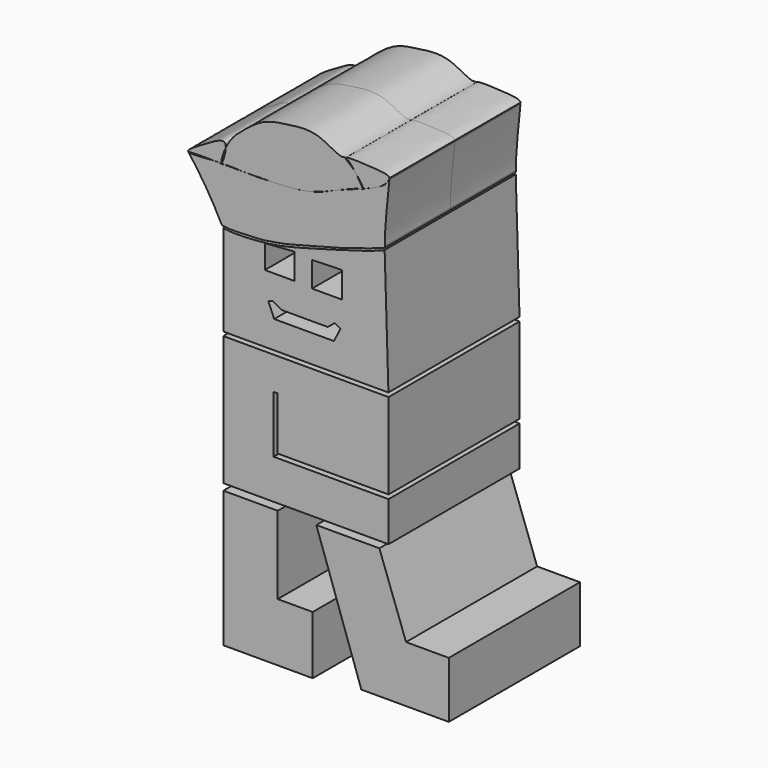
from build123d import *

# Parameters (mm, degrees)
F1_DEPTH      = 12.7
F1_DEPTH_BACK = 12.7


# Not quite as in the source:
# - a feature names something its author has since deleted; it is built from what else it names


with BuildPart() as f1:
    # F0 (on Front) → F1 (new body, two sides)
    with BuildSketch(Plane.XZ) as f1_sk:
        with BuildLine():
            add(Edge.make_bspline(
                [(-88.6765941978, 24.2591518909), (-88.676181883, 24.2590005668), (-88.6757689839, 24.2588493472), (-88.6753555008, 24.2586982322)],
                knots=[0, 0, 0, 0, 4.59815e-05, 4.59815e-05, 4.59815e-05, 4.59815e-05], degree=3))
            Line((-88.6765941978, 24.2591518909), (-88.6765941978, 10.1100709289))
            Line((-88.6765941978, 10.1100709289), (-63.0800493449, 10.1100709289))
            Line((-63.0800493449, 10.1100709289), (-63.6637075159, 29.3709366794))
            Line((-63.6637075159, 29.3709366794), (-64.1699039165, 29.1051819762))
            Line((-64.1699039165, 29.1051819762), (-64.7639196973, 28.9203976704))
            Line((-64.7639196973, 28.9203976704), (-65.5745303374, 28.6319091556))
            Line((-65.5745303374, 28.6319091556), (-67.1760400873, 28.1224887458))
            Line((-67.1760400873, 28.1224887458), (-68.6502717975, 27.6911423607))
            add(Edge.make_bspline(
                [(-70.894030415, 27.0381318624), (-70.1317684635, 27.256307302), (-69.3736818752, 27.476571284), (-68.6502717975, 27.6911423607)],
                knots=[0.2279945979, 0.2279945979, 0.2279945979, 0.2279945979, 0.247245534, 0.247245534, 0.247245534, 0.247245534], degree=3))
            add(Edge.make_bspline(
                [(-72.906285927, 26.4692383245), (-72.246354557, 26.6536394297), (-71.5685577228, 26.8450679274), (-70.894030415, 27.0381318624)],
                knots=[0.2109594015, 0.2109594015, 0.2109594015, 0.2109594015, 0.2279945979, 0.2279945979, 0.2279945979, 0.2279945979], degree=3))
            add(Edge.make_bspline(
                [(-74.0934775144, 26.1396786733), (-73.707677612, 26.2460726704), (-73.3103302266, 26.3563383796), (-72.906285927, 26.4692383245)],
                knots=[0.2005295684, 0.2005295684, 0.2005295684, 0.2005295684, 0.2109594015, 0.2109594015, 0.2109594015, 0.2109594015], degree=3))
            Line((-74.0934775144, 26.1396786733), (-75.0365182757, 25.8767232299))
            Line((-75.0365182757, 25.8767232299), (-75.7828429341, 25.6783552468))
            add(Edge.make_bspline(
                [(-76.5956836697, 25.4603034028), (-76.3368763961, 25.5291025193), (-76.0665517581, 25.6016964009), (-75.7828429341, 25.6783552468)],
                knots=[0.1756550657, 0.1756550657, 0.1756550657, 0.1756550657, 0.1843973599, 0.1843973599, 0.1843973599, 0.1843973599], degree=3))
            add(Edge.make_bspline(
                [(-77.3195936734, 25.2701518586), (-77.0880330237, 25.3301143771), (-76.8473015317, 25.3934154581), (-76.5956836697, 25.4603034028)],
                knots=[0.1671556239, 0.1671556239, 0.1671556239, 0.1671556239, 0.1756550657, 0.1756550657, 0.1756550657, 0.1756550657], degree=3))
            add(Edge.make_bspline(
                [(-78.2819622434, 25.0277422611), (-77.9772068237, 25.1019241231), (-77.6582053854, 25.1824685192), (-77.3195936734, 25.2701518586)],
                knots=[0.154726869, 0.154726869, 0.154726869, 0.154726869, 0.1671556239, 0.1671556239, 0.1671556239, 0.1671556239], degree=3))
            add(Edge.make_bspline(
                [(-79.7086635234, 24.7069066365), (-79.2560431416, 24.7986404801), (-78.7886960811, 24.9043959408), (-78.2819622434, 25.0277422611)],
                knots=[0.1340608848, 0.1340608848, 0.1340608848, 0.1340608848, 0.154726869, 0.154726869, 0.154726869, 0.154726869], degree=3))
            add(Edge.make_bspline(
                [(-80.8770336189, 24.4963051116), (-80.4878603762, 24.557399363), (-80.1038758883, 24.6268078368), (-79.7086635234, 24.7069066365)],
                knots=[0.1160160667, 0.1160160667, 0.1160160667, 0.1160160667, 0.1340608848, 0.1340608848, 0.1340608848, 0.1340608848], degree=3))
            Line((-80.8770336189, 24.4963051116), (-80.9098272944, 24.4904190618))
            Line((-80.9098272944, 24.4904190618), (-81.33696908, 24.4221940953))
            Line((-81.33696908, 24.4221940953), (-82.0637136126, 24.3332062233))
            Line((-82.0637136126, 24.3332062233), (-82.8794404293, 24.2501490134))
            Line((-82.8794404293, 24.2501490134), (-83.6002468491, 24.1937909592))
            Line((-83.6002468491, 24.1937909592), (-83.8359130376, 24.1790783462))
            add(Edge.make_bspline(
                [(-84.4445790934, 24.1410793947), (-84.2406040529, 24.1525204663), (-84.0370967315, 24.1652457772), (-83.8359130376, 24.1790783462)],
                knots=[0.0668457733, 0.0668457733, 0.0668457733, 0.0668457733, 0.0744285702, 0.0744285702, 0.0744285702, 0.0744285702], degree=3))
            Line((-84.4445790934, 24.1410793947), (-85.147680285, 24.0971848685))
            Line((-85.147680285, 24.0971848685), (-85.6315054246, 24.0900506289))
            add(Edge.make_bspline(
                [(-86.6028345544, 24.0757279031), (-86.2940429361, 24.0752792341), (-85.9672821173, 24.0803380751), (-85.6315054246, 24.0900506289)],
                knots=[0.0392199906, 0.0392199906, 0.0392199906, 0.0392199906, 0.0520326334, 0.0520326334, 0.0520326334, 0.0520326334], degree=3))
            add(Edge.make_bspline(
                [(-87.4198373818, 24.0923570373), (-87.1684176734, 24.0814558229), (-86.8935919097, 24.0761503687), (-86.6028345544, 24.0757279031)],
                knots=[0.0271556406, 0.0271556406, 0.0271556406, 0.0271556406, 0.0392199906, 0.0392199906, 0.0392199906, 0.0392199906], degree=3))
            add(Edge.make_bspline(
                [(-88.0641563934, 24.1389165741), (-87.8745442647, 24.1179875567), (-87.6576624685, 24.1026688074), (-87.4198373818, 24.0923570373)],
                knots=[0.0157436273, 0.0157436273, 0.0157436273, 0.0157436273, 0.0271556406, 0.0271556406, 0.0271556406, 0.0271556406], degree=3))
            add(Edge.make_bspline(
                [(-88.5565382268, 24.2221505155), (-88.4259838036, 24.1880082148), (-88.2595489318, 24.1604836219), (-88.0641563934, 24.1389165741)],
                knots=[0.0039837136, 0.0039837136, 0.0039837136, 0.0039837136, 0.0157436273, 0.0157436273, 0.0157436273, 0.0157436273], degree=3))
            add(Edge.make_bspline(
                [(-88.6359078797, 24.2451631992), (-88.6111654233, 24.237180281), (-88.5846857461, 24.2295115917), (-88.5565382268, 24.2221505155)],
                knots=[0.0014482776, 0.0014482776, 0.0014482776, 0.0014482776, 0.0039837136, 0.0039837136, 0.0039837136, 0.0039837136], degree=3))
            Line((-88.6359078797, 24.2451631992), (-88.6737406254, 24.2561325431))
            Line((-88.6737406254, 24.2561325431), (-88.6753555008, 24.2586982322))
        make_face()
        Polygon((-82.2262391448, 20.598737523), (-82.2262391448, 24.2591518909), (-77.6218995452, 24.6051102877), (-77.6218995452, 20.598737523), align=None, mode=Mode.SUBTRACT)
        Polygon((-80.7911232114, 14.3798924983), (-81.6880688071, 16.5325701237), (-80.9705108404, 16.7717561126), (-79.6549841762, 15.994399786), (-72.4793970585, 15.994399786), (-71.4150190353, 16.8674312532), (-70.5061107874, 16.4129771292), (-71.5226531029, 14.3798924983), align=None, mode=Mode.SUBTRACT)
        Polygon((-74.9200507998, 20.4430520535), (-74.9200507998, 24.3614321552), (-70.2414959669, 24.4861954051), (-70.2414959669, 20.4478651285), align=None, mode=Mode.SUBTRACT)
    extrude(amount=F1_DEPTH)
    extrude(f1_sk.sketch, amount=-F1_DEPTH_BACK)


with BuildPart() as f1b:
    # F0 (on Front) → F1, piece 2 (new body, two sides)
    with BuildSketch(Plane.XZ) as f1_2_sk:
        with BuildLine():
            Line((-89.1806710013, 25.0642394208), (-88.8575675001, 24.5481938542))
            Line((-88.8575675001, 24.5481938542), (-87.680645287, 24.4102943689))
            Line((-87.680645287, 24.4102943689), (-86.5415930748, 24.4221594185))
            Line((-86.5415930748, 24.4221594185), (-85.2364301682, 24.4696196169))
            Line((-85.2364301682, 24.4696196169), (-83.563439548, 24.5289467275))
            Line((-83.563439548, 24.5289467275), (-82.4006572366, 24.6238671243))
            Line((-82.4006572366, 24.6238671243), (-81.1148583889, 24.827260524))
            Line((-81.1148583889, 24.827260524), (-80.175191164, 24.9782800674))
            Line((-80.175191164, 24.9782800674), (-78.8160189986, 25.246758014))
            Line((-78.8160189986, 25.246758014), (-77.2387161851, 25.6494730711))
            Line((-77.2387161851, 25.6494730711), (-75.208351016, 26.1864289641))
            Line((-75.208351016, 26.1864289641), (-73.3753862668, 26.6711798054))
            Line((-73.3753862668, 26.6711798054), (-70.5099925399, 27.4281390011))
            Line((-70.5099925399, 27.4281390011), (-68.3453977108, 28.0993320048))
            Line((-68.3453977108, 28.0993320048), (-65.8955350518, 28.871204704))
            Line((-65.8955350518, 28.871204704), (-63.6414005769, 29.6839251888))
            Line((-63.6414005769, 29.6839251888), (-63.6204607901, 29.9628862484))
            add(Edge.make_bspline(
                [(-63.6204607901, 29.9628862484), (-63.7690930896, 31.4681703482), (-63.0734122524, 37.8136935829), (-62.9346598656, 39.1672787688)],
                knots=[0.3407241659, 0.3407241659, 0.3407241659, 0.3407241659, 0.4433037601, 0.4433037601, 0.4433037601, 0.4433037601], degree=3))
            add(Edge.make_bspline(
                [(-62.9346598656, 39.1672787688), (-62.99116387, 39.0074353898), (-63.1238176876, 38.8255438406), (-63.3057207132, 38.6381461886)],
                knots=[0.3858068106, 0.3858068106, 0.3858068106, 0.3858068106, 0.4313082922, 0.4313082922, 0.4313082922, 0.4313082922], degree=3))
            add(Edge.make_bspline(
                [(-63.3057207132, 38.6381461886), (-63.591865805, 38.282485153), (-64.0700130065, 37.9519174396), (-64.6626520258, 37.6396269978)],
                knots=[0.4854255945, 0.4854255945, 0.4854255945, 0.4854255945, 0.5132501123, 0.5132501123, 0.5132501123, 0.5132501123], degree=3))
            add(Edge.make_bspline(
                [(-64.6626520258, 37.6396269978), (-64.9284082914, 37.492687811), (-65.1932928871, 37.3699325807), (-65.4429785447, 37.2647073069)],
                knots=[0.5161566053, 0.5161566053, 0.5161566053, 0.5161566053, 0.5606076079, 0.5606076079, 0.5606076079, 0.5606076079], degree=3))
            add(Edge.make_bspline(
                [(-65.4429785447, 37.2647073069), (-65.8563362693, 37.081501475), (-66.3008735293, 36.9041305775), (-66.7586636583, 36.7310181908)],
                knots=[0.5246441776, 0.5246441776, 0.5246441776, 0.5246441776, 0.5417236467, 0.5417236467, 0.5417236467, 0.5417236467], degree=3))
            add(Edge.make_bspline(
                [(-66.7586636583, 36.7310181908), (-66.8712838712, 36.6647105624), (-66.9239643529, 36.6009277441), (-66.9972679395, 36.641578996)],
                knots=[0.6640545001, 0.6640545001, 0.6640545001, 0.6640545001, 0.7134494162, 0.7134494162, 0.7134494162, 0.7134494162], degree=3))
            add(Edge.make_bspline(
                [(-66.9972679395, 36.641578996), (-67.0125383393, 36.5119331388), (-67.1907492056, 36.5231425104), (-67.4698356723, 36.4682586449)],
                knots=[0.5691718068, 0.5691718068, 0.5691718068, 0.5691718068, 0.5952228955, 0.5952228955, 0.5952228955, 0.5952228955], degree=3))
            add(Edge.make_bspline(
                [(-67.4698356723, 36.4682586449), (-68.3929391768, 36.1336333741), (-69.5493172224, 35.7381934495), (-70.5194605701, 35.3447298383), (-70.696805174, 35.2710997008)],
                knots=[0.5504682125, 0.5504682125, 0.5504682125, 0.5504682125, 0.5842531146, 0.5920722335, 0.5920722335, 0.5920722335, 0.5920722335], degree=3))
            add(Edge.make_bspline(
                [(-70.696805174, 35.2710997008), (-70.908839023, 35.1812273665), (-71.1199071334, 35.0913269662), (-71.3269268074, 35.0033066073)],
                knots=[0.6590265835, 0.6590265835, 0.6590265835, 0.6590265835, 0.6698079497, 0.6698079497, 0.6698079497, 0.6698079497], degree=3))
            add(Edge.make_bspline(
                [(-71.3269268074, 35.0033066073), (-72.6834973217, 34.4164241105), (-73.8406974955, 33.8702485293), (-75.6439072937, 33.4965059757)],
                knots=[0.6016179317, 0.6016179317, 0.6016179317, 0.6016179317, 0.6649272201, 0.6649272201, 0.6649272201, 0.6649272201], degree=3))
            add(Edge.make_bspline(
                [(-75.6439072937, 33.4965059757), (-76.405580982, 33.3335271633), (-77.2236332809, 33.2252564375), (-78.0591693269, 33.1491839613)],
                knots=[0.7483248245, 0.7483248245, 0.7483248245, 0.7483248245, 0.7877632518, 0.7877632518, 0.7877632518, 0.7877632518], degree=3))
            add(Edge.make_bspline(
                [(-78.0591693269, 33.1491839613), (-78.9314375594, 33.0688250448), (-79.9140408829, 33.0151128871), (-80.9525646713, 32.9802233287)],
                knots=[0.6892796952, 0.6892796952, 0.6892796952, 0.6892796952, 0.7121210529, 0.7121210529, 0.7121210529, 0.7121210529], degree=3))
            add(Edge.make_bspline(
                [(-80.9525646713, 32.9802233287), (-82.6104794056, 32.9162984037), (-84.1581399366, 32.8778860173), (-85.6189520723, 32.9232138611)],
                knots=[0.8331267481, 0.8331267481, 0.8331267481, 0.8331267481, 0.912449519, 0.912449519, 0.912449519, 0.912449519], degree=3))
            add(Edge.make_bspline(
                [(-85.6189520723, 32.9232138611), (-86.594573022, 32.9259699322), (-87.5521865291, 32.9348252964), (-88.4524292433, 32.944119984)],
                knots=[0.744974607, 0.744974607, 0.744974607, 0.744974607, 0.7654790219, 0.7654790219, 0.7654790219, 0.7654790219], degree=3))
            add(Edge.make_bspline(
                [(-88.4524292433, 32.944119984), (-88.7063087421, 32.9022333853), (-88.8776467113, 32.8279592391), (-88.9438291909, 32.9492656946)],
                knots=[0.9742592774, 0.9742592774, 0.9742592774, 0.9742592774, 1, 1, 1, 1], degree=3))
            add(Edge.make_bspline(
                [(-88.9438291909, 32.9492656946), (-89.0352585897, 32.8295840724), (-89.0788010883, 32.9176528435), (-89.3225391675, 32.9532516827)],
                knots=[0.6558803024, 0.6558803024, 0.6558803024, 0.6558803024, 0.7317333454, 0.7317333454, 0.7317333454, 0.7317333454], degree=3))
            add(Edge.make_bspline(
                [(-89.3225391675, 32.9532516827), (-89.5940767888, 32.9560898012), (-89.8585710886, 32.9587851097), (-90.1147749683, 32.9611582906)],
                knots=[0.7722377312, 0.7722377312, 0.7722377312, 0.7722377312, 0.7787258229, 0.7787258229, 0.7787258229, 0.7787258229], degree=3))
            add(Edge.make_bspline(
                [(-90.1147749683, 32.9611582906), (-91.4362647143, 32.8979274564), (-93.6540192513, 32.6111194745), (-94.0586850047, 32.8551717103)],
                knots=[0.7863292069, 0.7863292069, 0.7863292069, 0.7863292069, 1, 1, 1, 1], degree=3))
            Line((-94.0586850047, 32.8551717103), (-93.7775747638, 32.4061957846))
            add(Edge.make_bspline(
                [(-93.7775747638, 32.4061957846), (-92.6941800923, 31.2024334146), (-89.8309867411, 26.6093738398), (-89.1806710013, 25.0642394208)],
                knots=[0.858322558, 0.858322558, 0.858322558, 0.858322558, 0.9647554778, 0.9647554778, 0.9647554778, 0.9647554778], degree=3))
        make_face()
    extrude(amount=F1_DEPTH)
    extrude(f1_2_sk.sketch, amount=-F1_DEPTH_BACK)


with BuildPart() as f1c:
    # F0 (on Front) → F1, piece 3 (new body, two sides)
    with BuildSketch(Plane.XZ) as f1_3_sk:
        Polygon((-63.0613416433, 9.4927120954), (-88.6765941978, 9.4927120954), (-88.6765941978, 0), (-88.6765941978, -10.5822533369), (-63.0613416433, -10.5822533369), (-63.0613416433, -4.4350544922), (-80.8818116784, -4.4350544922), (-80.8818116784, 4.4147078879), (-80.3020894527, 4.4147078879), (-80.3020894527, -3.7941283081), (-63.0613416433, -3.7941283081), align=None)
    extrude(amount=F1_DEPTH)
    extrude(f1_3_sk.sketch, amount=-F1_DEPTH_BACK)


with BuildPart() as f1d:
    # F0 (on Front) → F1, piece 4 (new body, two sides)
    with BuildSketch(Plane.XZ) as f1_4_sk:
        with BuildLine():
            add(Edge.make_bspline(
                [(-94.0586850047, 32.8551717103), (-94.4654065338, 33.1004637757), (-91.5178597494, 34.7172704345), (-88.4386957073, 36.6762673441), (-88.2852047026, 35.5322981305), (-88.2893016676, 35.317583748)],
                knots=[0, 0, 0, 0, 0.2147562796, 0.444264687, 0.4880842191, 0.4880842191, 0.4880842191, 0.4880842191], degree=3))
            add(Edge.make_bspline(
                [(-90.1147749683, 32.9611582906), (-92.2185943193, 32.9806456768), (-93.7634005143, 32.9784123854), (-94.0586850047, 32.8551717103)],
                knots=[0.7787258229, 0.7787258229, 0.7787258229, 0.7787258229, 0.8320028174, 0.8320028174, 0.8320028174, 0.8320028174], degree=3))
            add(Edge.make_bspline(
                [(-89.3225391675, 32.9532516827), (-89.4979716868, 32.9788742447), (-89.7771159455, 32.9773146488), (-90.1147749683, 32.9611582906)],
                knots=[0.7317333454, 0.7317333454, 0.7317333454, 0.7317333454, 0.7863292069, 0.7863292069, 0.7863292069, 0.7863292069], degree=3))
            add(Edge.make_bspline(
                [(-88.9438291909, 32.9492656946), (-89.0714727093, 32.9506129158), (-89.1977497163, 32.9519473801), (-89.3225391675, 32.9532516827)],
                knots=[0.7692560251, 0.7692560251, 0.7692560251, 0.7692560251, 0.7722377312, 0.7722377312, 0.7722377312, 0.7722377312], degree=3))
            add(Edge.make_bspline(
                [(-88.9438291909, 32.9492656946), (-89.0819981393, 33.2025167887), (-88.7618492252, 34.3082015855), (-88.2893016589, 35.3175837458)],
                knots=[0, 0, 0, 0, 0.0537388232, 0.0537388232, 0.0537388232, 0.0537388232], degree=3))
        make_face()
    extrude(amount=F1_DEPTH)
    extrude(f1_4_sk.sketch, amount=-F1_DEPTH_BACK)


with BuildPart() as f1e:
    # F0 (on Front) → F1, piece 5 (new body, two sides)
    with BuildSketch(Plane.XZ) as f1_5_sk:
        with BuildLine():
            add(Edge.make_bspline(
                [(-88.2893016589, 35.3175837458), (-88.1899717612, 35.5297567288), (-87.4282788512, 37.0229144843), (-85.6108289308, 38.5700062743), (-82.4464479, 41.1116553012), (-78.4456250447, 41.644345132), (-74.1132724556, 42.2162050244), (-70.5326189415, 39.6499089464), (-69.9159322613, 40.020232556), (-69.6954354644, 39.9633795023)],
                knots=[0.0537388232, 0.0537388232, 0.0537388232, 0.0537388232, 0.0650347692, 0.1348604038, 0.2069273895, 0.2800852866, 0.3577229921, 0.4305213633, 0.4616432126, 0.4616432126, 0.4616432126, 0.4616432126], degree=3))
            add(Edge.make_bspline(
                [(-88.2893016676, 35.317583748), (-88.3049899843, 34.495388012), (-88.7415763291, 33.2140158836), (-88.9438291909, 32.9492656946)],
                knots=[0.4880842191, 0.4880842191, 0.4880842191, 0.4880842191, 0.6558803024, 0.6558803024, 0.6558803024, 0.6558803024], degree=3))
            add(Edge.make_bspline(
                [(-88.4524292433, 32.944119984), (-88.6182578996, 32.9458321062), (-88.7821398929, 32.9475591352), (-88.9438291909, 32.9492656946)],
                knots=[0.7654790219, 0.7654790219, 0.7654790219, 0.7654790219, 0.7692560251, 0.7692560251, 0.7692560251, 0.7692560251], degree=3))
            add(Edge.make_bspline(
                [(-85.6189520723, 32.9232138611), (-86.7572436907, 32.9585341486), (-87.8428025932, 33.0446999322), (-88.4524292433, 32.944119984)],
                knots=[0.912449519, 0.912449519, 0.912449519, 0.912449519, 0.9742592774, 0.9742592774, 0.9742592774, 0.9742592774], degree=3))
            add(Edge.make_bspline(
                [(-80.9525646713, 32.9802233287), (-82.446311143, 32.9300404101), (-84.0557465065, 32.9187978983), (-85.6189520723, 32.9232138611)],
                knots=[0.7121210529, 0.7121210529, 0.7121210529, 0.7121210529, 0.744974607, 0.744974607, 0.744974607, 0.744974607], degree=3))
            add(Edge.make_bspline(
                [(-78.0591693269, 33.1491839613), (-79.0202329114, 33.0616826656), (-80.00442824, 33.0167810292), (-80.9525646713, 32.9802233287)],
                knots=[0.7877632518, 0.7877632518, 0.7877632518, 0.7877632518, 0.8331267481, 0.8331267481, 0.8331267481, 0.8331267481], degree=3))
            add(Edge.make_bspline(
                [(-75.6439072937, 33.4965059757), (-76.2263444498, 33.3757870498), (-77.0002283612, 33.2534476063), (-77.9100997071, 33.1629172061), (-78.0591693269, 33.1491839613)],
                knots=[0.6649272201, 0.6649272201, 0.6649272201, 0.6649272201, 0.685376134, 0.6892796952, 0.6892796952, 0.6892796952, 0.6892796952], degree=3))
            add(Edge.make_bspline(
                [(-71.3269268074, 35.0033066073), (-72.8345778324, 34.3622854825), (-74.1275122007, 33.8209759885), (-75.6439072937, 33.4965059757)],
                knots=[0.6698079497, 0.6698079497, 0.6698079497, 0.6698079497, 0.7483248245, 0.7483248245, 0.7483248245, 0.7483248245], degree=3))
            add(Edge.make_bspline(
                [(-70.696805174, 35.2710997008), (-70.9133101386, 35.1812109195), (-71.1223847401, 35.0917960429), (-71.3269268074, 35.0033066073)],
                knots=[0.5920722335, 0.5920722335, 0.5920722335, 0.5920722335, 0.6016179317, 0.6016179317, 0.6016179317, 0.6016179317], degree=3))
            add(Edge.make_bspline(
                [(-67.4698356723, 36.4682586449), (-68.1533674068, 36.3338384266), (-69.4419974553, 35.8029605303), (-70.696805174, 35.2710997008)],
                knots=[0.5952228955, 0.5952228955, 0.5952228955, 0.5952228955, 0.6590265835, 0.6590265835, 0.6590265835, 0.6590265835], degree=3))
            add(Edge.make_bspline(
                [(-66.9972679395, 36.641578996), (-67.1538562949, 36.5833678168), (-67.3116117825, 36.5256148479), (-67.4698356723, 36.4682586449)],
                knots=[0.5446773358, 0.5446773358, 0.5446773358, 0.5446773358, 0.5504682125, 0.5504682125, 0.5504682125, 0.5504682125], degree=3))
            add(Edge.make_bspline(
                [(-66.9972679395, 36.641578996), (-67.1899806678, 36.7484498059), (-67.5252293414, 37.5771134318), (-68.0491964268, 38.2991926754)],
                knots=[0.7134494162, 0.7134494162, 0.7134494162, 0.7134494162, 0.8433070328, 0.8433070328, 0.8433070328, 0.8433070328], degree=3))
            add(Edge.make_bspline(
                [(-68.3385133528, 38.6603101822), (-68.243943305, 38.5433232102), (-68.1464445488, 38.421940349), (-68.0491964092, 38.2991926535)],
                knots=[0.5120070004, 0.5120070004, 0.5120070004, 0.5120070004, 0.5206749385, 0.5206749385, 0.5206749385, 0.5206749385], degree=3))
            add(Edge.make_bspline(
                [(-68.3385133743, 38.6603102088), (-68.9490155106, 39.3428137328), (-69.7696484591, 39.7582813111), (-69.6954354644, 39.9633795023)],
                knots=[0.8657866504, 0.8657866504, 0.8657866504, 0.8657866504, 1, 1, 1, 1], degree=3))
        make_face()
    extrude(amount=F1_DEPTH)
    extrude(f1_5_sk.sketch, amount=-F1_DEPTH_BACK)


with BuildPart() as f1f:
    # F0 (on Front) → F1, piece 6 (new body, two sides)
    with BuildSketch(Plane.XZ) as f1_6_sk:
        with BuildLine():
            add(Edge.make_bspline(
                [(-69.6954354644, 39.9633795023), (-69.5928784024, 40.2468105639), (-66.0746656855, 40.0170166953), (-63.0605680011, 39.9117810844), (-62.9163475392, 39.4130423093)],
                knots=[0, 0, 0, 0, 0.1854732699, 0.3602240374, 0.3602240374, 0.3602240374, 0.3602240374], degree=3))
            add(Edge.make_bspline(
                [(-69.6954354644, 39.9633795023), (-69.3386104631, 39.8713754858), (-68.8879988155, 39.3400459114), (-68.3385133528, 38.6603101822)],
                knots=[0.4616432126, 0.4616432126, 0.4616432126, 0.4616432126, 0.5120070004, 0.5120070004, 0.5120070004, 0.5120070004], degree=3))
            add(Edge.make_bspline(
                [(-68.0491964268, 38.2991926754), (-68.13990023, 38.4241916219), (-68.2362593542, 38.5459965562), (-68.3385133743, 38.6603102088)],
                knots=[0.8433070328, 0.8433070328, 0.8433070328, 0.8433070328, 0.8657866504, 0.8657866504, 0.8657866504, 0.8657866504], degree=3))
            add(Edge.make_bspline(
                [(-68.0491964268, 38.2991926754), (-67.5050958349, 37.6124227898), (-66.9688404686, 36.8829285274), (-66.9972679395, 36.641578996)],
                knots=[0.5206749385, 0.5206749385, 0.5206749385, 0.5206749385, 0.5691718068, 0.5691718068, 0.5691718068, 0.5691718068], degree=3))
            add(Edge.make_bspline(
                [(-66.7586636583, 36.7310181908), (-66.8378329644, 36.7010804821), (-66.9173986313, 36.671270135), (-66.9972679395, 36.641578996)],
                knots=[0.5417236467, 0.5417236467, 0.5417236467, 0.5417236467, 0.5446773358, 0.5446773358, 0.5446773358, 0.5446773358], degree=3))
            add(Edge.make_bspline(
                [(-65.4429785447, 37.2647073069), (-66.0240499219, 37.0198258212), (-66.5228051543, 36.8698850748), (-66.7586636583, 36.7310181908)],
                knots=[0.5606076079, 0.5606076079, 0.5606076079, 0.5606076079, 0.6640545001, 0.6640545001, 0.6640545001, 0.6640545001], degree=3))
            add(Edge.make_bspline(
                [(-64.6626520258, 37.6396269978), (-64.90533611, 37.511744902), (-65.1672191034, 37.3869276861), (-65.4429785447, 37.2647073069)],
                knots=[0.5132501123, 0.5132501123, 0.5132501123, 0.5132501123, 0.5246441776, 0.5246441776, 0.5246441776, 0.5246441776], degree=3))
            add(Edge.make_bspline(
                [(-63.3057207132, 38.6381461886), (-63.6449220822, 38.2886987844), (-64.1553750352, 37.9201053087), (-64.6626520258, 37.6396269978)],
                knots=[0.4313082922, 0.4313082922, 0.4313082922, 0.4313082922, 0.5161566053, 0.5161566053, 0.5161566053, 0.5161566053], degree=3))
            add(Edge.make_bspline(
                [(-62.9163475392, 39.4130423093), (-62.9376753226, 39.3478946261), (-63.030672716, 38.9852317508), (-63.2997854361, 38.6455233789), (-63.3057207132, 38.6381461886)],
                knots=[0.4588879418, 0.4588879418, 0.4588879418, 0.4588879418, 0.484848453, 0.4854255945, 0.4854255945, 0.4854255945, 0.4854255945], degree=3))
        make_face()
    extrude(amount=F1_DEPTH)
    extrude(f1_6_sk.sketch, amount=-F1_DEPTH_BACK)


with BuildPart() as f1g:
    # F0 (on Front) → F1, piece 7 (new body, two sides)
    with BuildSketch(Plane.XZ) as f1_7_sk:
        Polygon((-80.2386254072, -11.6022033617), (-88.6765941978, -11.6022033617), (-88.6765941978, -32.6971188188), (-74.814222753, -32.6971188188), (-74.814222753, -23.6564408988), (-80.2386254072, -23.6564408988), align=None)
    extrude(amount=F1_DEPTH)
    extrude(f1_7_sk.sketch, amount=-F1_DEPTH_BACK)


with BuildPart() as f1h:
    # F0 (on Front) → F1, piece 8 (new body, two sides)
    with BuildSketch(Plane.XZ) as f1_8_sk:
        Polygon((-60.349136591, -23.053728044), (-64.479433, -11.6022033617), (-71.6499835253, -11.6022033617), (-74.2485448718, -11.6022033617), (-67.2803223133, -31.793050468), (-53.719304502, -31.793050468), (-53.719304502, -23.053728044), align=None)
    extrude(amount=F1_DEPTH)
    extrude(f1_8_sk.sketch, amount=-F1_DEPTH_BACK)


solid = Compound([f1.part, f1b.part, f1c.part, f1d.part, f1e.part, f1f.part, f1g.part, f1h.part])
